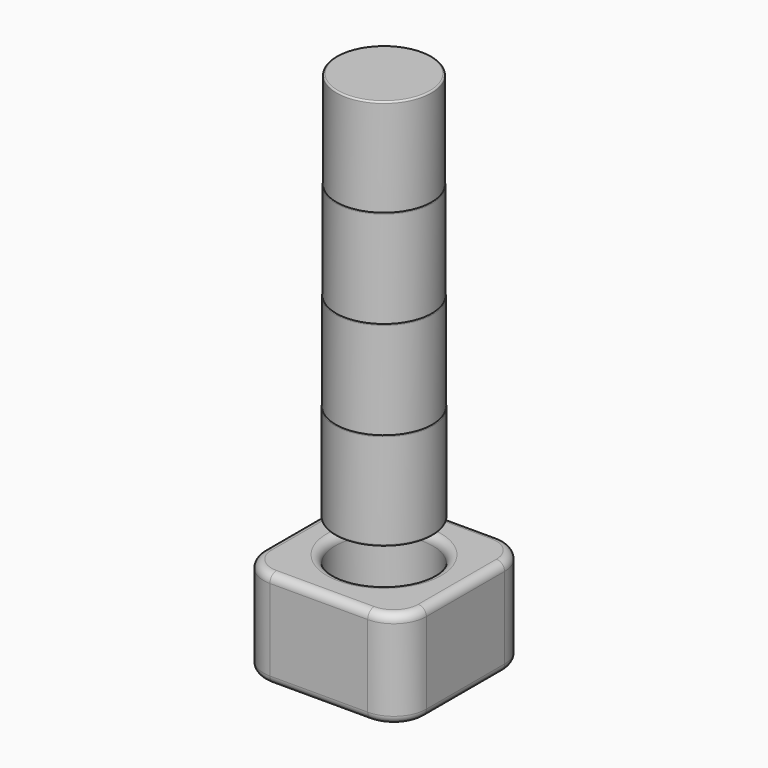
from build123d import *

# Parameters (mm, degrees)
F0_W     = 10
F0_H     = 10
F0_R     = 3
F1_DEPTH = 6
F2_R     = 0.5
F3_R     = 2
F4_R     = 0.5


# Not quite as in the source:
# - a fillet or chamfer that OpenCascade refuses, or shapes differently, is made with other operations: its cross-section is extruded or revolved along the edge and cut away or added


with BuildPart() as f1:
    # F0 (on Top) → F1 (new body)
    with BuildSketch(Plane.XY):
        Rectangle(F0_W, F0_H)
        Circle(F0_R, mode=Mode.SUBTRACT)
    extrude(amount=-F1_DEPTH)

    # F2
    f2_edges = [f1.edges().sort_by_distance(p)[0] for p in [
        (-3, 0, -6),
        (-3, 0, 0),
    ]]
    fillet(f2_edges, radius=F2_R)

    # F3
    f3_edges = [f1.edges().sort_by_distance(p)[0] for p in [
        (-5, -5, -3),
        (5, -5, -3),
        (-5, 5, -3),
        (5, 5, -3),
    ]]
    fillet(f3_edges, radius=F3_R)

    # F4
    f4_edges = [f1.edges().sort_by_distance(p)[0] for p in [
        (-4.414214, -4.414214, -6),
        (-4.414214, -4.414214, 0),
        (5, 0, 0),
        (4.414214, -4.414214, 0),
        (4.414214, 4.414214, 0),
        (0, -5, 0),
        (0, 5, 0),
        (-4.414214, 4.414214, 0),
        (-5, 0, 0),
        (5, 0, -6),
        (4.414214, -4.414214, -6),
        (4.414214, 4.414214, -6),
        (0, -5, -6),
        (0, 5, -6),
        (-4.414214, 4.414214, -6),
        (-5, 0, -6),
    ]]
    fillet(f4_edges, radius=F4_R)


with BuildPart() as f6:
    # F5 (on Front) → F6 (revolve)
    with BuildSketch(Plane.XZ):
        Polygon((0, 2), (0, 26), (-2.925, 26), (-2.925, 20), (-2.95, 20), (-2.95, 14), (-2.975, 14), (-2.975, 8), (-3, 8), (-3, 2), align=None)
    revolve(axis=Axis((0, 0, 14), (0, 0, -1)))

    # F7: fillet of radius 0.1 on 5 edges, made by hand

    # F7_s1 → F7_t2 (revolve, cut)
    with BuildSketch(Plane.XZ):
        with BuildLine():
            ThreePointArc((-2.925, 20), (-2.9435414347, 19.9692115563), (-2.95, 19.9338562172))
            Line((-2.95, 19.9338562172), (-2.95, 20))
            Line((-2.95, 20), (-2.925, 20))
        make_face()
    revolve(axis=Axis((0, 0, 20), (0, 0, -1)), mode=Mode.SUBTRACT)

    # F7_s3 → F7_t4 (revolve, cut)
    with BuildSketch(Plane.XZ):
        with BuildLine():
            ThreePointArc((-2.95, 14), (-2.9685414347, 13.9692115563), (-2.975, 13.9338562172))
            Line((-2.975, 13.9338562172), (-2.975, 14))
            Line((-2.975, 14), (-2.95, 14))
        make_face()
    revolve(axis=Axis((0, 0, 14), (0, 0, -1)), mode=Mode.SUBTRACT)

    # F7_s5 → F7_t6 (revolve, cut)
    with BuildSketch(Plane.XZ):
        with BuildLine():
            ThreePointArc((-2.975, 8), (-2.9935414347, 7.9692115563), (-3, 7.9338562172))
            Line((-3, 7.9338562172), (-3, 8))
            Line((-3, 8), (-2.975, 8))
        make_face()
    revolve(axis=Axis((0, 0, 8), (0, 0, -1)), mode=Mode.SUBTRACT)

    # F7_s7 → F7_t8 (revolve, cut)
    with BuildSketch(Plane.XZ):
        with BuildLine():
            ThreePointArc((-2.825, 26), (-2.8957106781, 25.9707106781), (-2.925, 25.9))
            Line((-2.925, 25.9), (-2.925, 26))
            Line((-2.925, 26), (-2.825, 26))
        make_face()
    revolve(axis=Axis((0, 0, 26), (0, 0, -1)), mode=Mode.SUBTRACT)

    # F7_s9 → F7_t10 (revolve, cut)
    with BuildSketch(Plane.XZ):
        with BuildLine():
            ThreePointArc((-3, 2.1), (-2.9707106781, 2.0292893219), (-2.9, 2))
            Line((-2.9, 2), (-3, 2))
            Line((-3, 2), (-3, 2.1))
        make_face()
    revolve(axis=Axis((0, 0, 2), (0, 0, -1)), mode=Mode.SUBTRACT)


solid = Compound([f1.part, f6.part])
